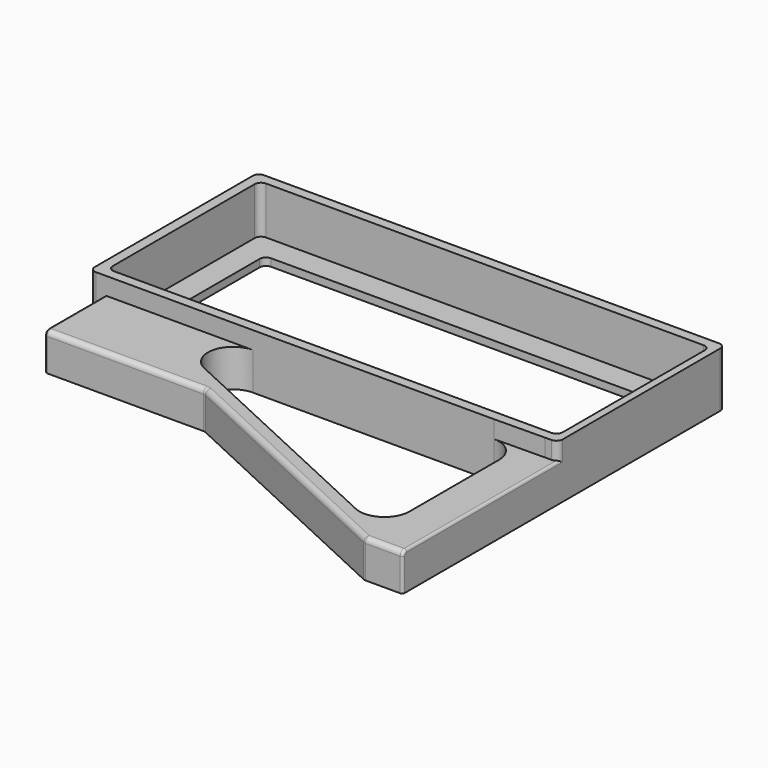
from build123d import *

# Parameters (mm, degrees)
F1_DEPTH     = 22
F2_DEPTH     = 3
F3_DEPTH     = 15
F0_W         = 15
F0_H         = 30
F4_DEPTH     = 15
F5_R         = 2
F6_T1_DEPTH  = 111.1292207426
F6_T3_DEPTH  = 68.4264144678
F6_T5_DEPTH  = 14.1054111362
F6_T10_DEPTH = 2
F6_T14_ANGLE = 24.9330990778
F7_R         = 1
F8_R         = 1
F9_DEPTH     = 5


# Not quite as in the source:
# - a fillet or chamfer that OpenCascade refuses, or shapes differently, is made with other operations: its cross-section is extruded or revolved along the edge and cut away or added
# - a feature names something its author has since deleted; it is built from what else it names


with BuildPart() as f1:
    # F0 (on Top) → F1 (new body)
    with BuildSketch(Plane.XY):
        with BuildLine():
            ThreePointArc((93, 77.5), (92.267766953, 79.267766953), (90.5, 80))
            Line((90.5, 80), (36.5, 80))
            Line((36.5, 80), (24.5, 80))
            Line((24.5, 80), (19, 80))
            Line((19, 80), (-7, 80))
            Line((-7, 80), (-12.5, 80))
            Line((-12.5, 80), (-24.5, 80))
            Line((-24.5, 80), (-74, 80))
            Line((-74, 80), (-91.5, 80))
            ThreePointArc((-91.5, 80), (-93.267766953, 79.267766953), (-94, 77.5))
            Line((-94, 77.5), (-94, 76))
            Line((-94, 76), (-94, 0))
            Line((-94, 0), (-94, -1.5))
            ThreePointArc((-94, -1.5), (-93.267766953, -3.267766953), (-91.5, -4))
            Line((-91.5, -4), (-88, -4))
            Line((-88, -4), (-73, -4))
            Line((-73, -4), (-28.6959191337, -4))
            Line((-28.6959191337, -4), (67.7072161436, -4))
            Line((67.7072161436, -4), (88, -3.7670015892))
            Line((88, -3.7670015892), (90.5, -3.7670015892))
            ThreePointArc((90.5, -3.7670015892), (92.267766953, -3.0347685421), (93, -1.2670015892))
            Line((93, -1.2670015892), (93, 0))
            Line((93, 0), (93, 76))
            Line((93, 76), (93, 77.5))
        make_face()
        with BuildLine():
            ThreePointArc((90, 2.5), (89.267766953, 0.732233047), (87.5, 0))
            Line((87.5, 0), (-87.5, 0))
            ThreePointArc((-87.5, 0), (-89.267766953, 0.732233047), (-90, 2.5))
            Line((-90, 2.5), (-90, 73.5))
            ThreePointArc((-90, 73.5), (-89.267766953, 75.267766953), (-87.5, 76))
            Line((-87.5, 76), (87.5, 76))
            ThreePointArc((87.5, 76), (89.267766953, 75.267766953), (90, 73.5))
            Line((90, 73.5), (90, 2.5))
        make_face(mode=Mode.SUBTRACT)
    extrude(amount=F1_DEPTH)

    # F0 (on Top) → F2 (join)
    with BuildSketch(Plane.XY):
        with BuildLine():
            Line((-87.5, 0), (87.5, 0))
            ThreePointArc((87.5, 0), (89.267766953, 0.732233047), (90, 2.5))
            Line((90, 2.5), (90, 73.5))
            ThreePointArc((90, 73.5), (89.267766953, 75.267766953), (87.5, 76))
            Line((87.5, 76), (-87.5, 76))
            ThreePointArc((-87.5, 76), (-89.267766953, 75.267766953), (-90, 73.5))
            Line((-90, 73.5), (-90, 2.5))
            ThreePointArc((-90, 2.5), (-89.267766953, 0.732233047), (-87.5, 0))
        make_face()
        with BuildLine():
            Line((-77.5, 66), (77.5, 66))
            ThreePointArc((77.5, 66), (79.267766953, 65.267766953), (80, 63.5))
            Line((80, 63.5), (80, 12.5))
            ThreePointArc((80, 12.5), (79.267766953, 10.732233047), (77.5, 10))
            Line((77.5, 10), (-77.5, 10))
            ThreePointArc((-77.5, 10), (-79.267766953, 10.732233047), (-80, 12.5))
            Line((-80, 12.5), (-80, 63.5))
            ThreePointArc((-80, 63.5), (-79.267766953, 65.267766953), (-77.5, 66))
        make_face(mode=Mode.SUBTRACT)
    extrude(amount=F2_DEPTH)

    # F0 (on Top) → F3 (join)
    with BuildSketch(Plane.XY):
        with BuildLine():
            Line((93, -81.2670015892), (93, -1.2670015892))
            ThreePointArc((93, -1.2670015892), (92.267766953, -3.0347685421), (90.5, -3.7670015892))
            Line((90.5, -3.7670015892), (88, -3.7670015892))
            Line((88, -3.7670015892), (67.7072161436, -4))
            ThreePointArc((67.7072161436, -4), (74.7782839555, -6.9289321881), (77.7072161436, -14))
            Line((77.7072161436, -14), (77.7072161436, -58.7379819401))
            ThreePointArc((77.7072161436, -58.7379819401), (73.0879609173, -67.1669549309), (63.4976990076, -67.8088124137))
            Line((63.4976990076, -67.8088124137), (-32.9054362697, -23.0708304737))
            ThreePointArc((-32.9054362697, -23.0708304737), (-38.4608642113, -11.8445771571), (-28.6959191337, -4))
            Line((-28.6959191337, -4), (-73, -4))
            Line((-73, -4), (-73, -34))
            Line((-73, -34), (-24.5735855322, -34))
            ThreePointArc((-24.5735855322, -34), (-24.033911544, -34.0589444934), (-23.5196862036, -34.2329984108))
            Line((-23.5196862036, -34.2329984108), (77.653316815, -81.2670015892))
            Line((77.653316815, -81.2670015892), (93, -81.2670015892))
        make_face()
    extrude(amount=F3_DEPTH)

    # F0 (on Top) → F4 (join)
    with BuildSketch(Plane.XY):
        with Locations((-80.5, -19)):
            Rectangle(F0_W, F0_H)
    extrude(amount=F4_DEPTH)

    # F5
    f5_edges = [f1.edges().sort_by_distance(p)[0] for p in [
        (85.326658, -81.267002, 15),
    ]]
    fillet(f5_edges, radius=F5_R)

    # F6: fillet of radius 2 on 4 edges, made by hand

    # F6_s2 → F6_t1 (cut)
    with BuildSketch(Plane(origin=(-6.2536714965, 2.9072499211, 0), x_dir=(0, 0, 1), z_dir=(0.9068006357, -0.4215597314, 0))):
        with BuildLine():
            ThreePointArc((15, 38.9574573188), (14.4142135624, 40.3716708812), (13, 40.9574573188))
            Line((13, 40.9574573188), (15, 40.9574573188))
            Line((15, 40.9574573188), (15, 38.9574573188))
        make_face()
    extrude(amount=F6_T1_DEPTH, mode=Mode.SUBTRACT)

    # F6_s4 → F6_t3 (cut)
    with BuildSketch(Plane.YZ.offset(-93)):
        with BuildLine():
            ThreePointArc((-32, 15), (-33.4142135624, 14.4142135624), (-34, 13))
            Line((-34, 13), (-34, 15))
            Line((-34, 15), (-32, 15))
        make_face()
    extrude(amount=F6_T3_DEPTH, mode=Mode.SUBTRACT)

    # F6_s6 → F6_t5 (cut)
    with BuildSketch(Plane.XY.offset(-1.1054111362)):
        with BuildLine():
            ThreePointArc((77.2523618067, -81.0806028605), (77.6637420789, -81.2198459945), (78.0954812695, -81.2670015892))
            Line((78.0954812695, -81.2670015892), (77.653316815, -81.2670015892))
            Line((77.653316815, -81.2670015892), (77.2523618067, -81.0806028605))
        make_face()
    extrude(amount=F6_T5_DEPTH, mode=Mode.SUBTRACT)


with BuildPart() as f6_tool8:
    # F6_s9 → F6_t10 (new body)
    with BuildSketch(Plane.XY.offset(13)):
        Polygon((78.0954812695, -79.2670015892), (78.0954812695, -81.2670015892), (77.653316815, -81.2670015892), (77.2523618067, -81.0806028605), align=None)
    extrude(amount=F6_T10_DEPTH)

    # F6_s11 → F6_t12 (revolve, cut)
    with BuildSketch(Plane(origin=(78.0954812695, -79.2670015892, 13), x_dir=(0.2158695953, 0.9764222027, 0), z_dir=(0.9764222027, -0.2158695953, 0))):
        with BuildLine():
            ThreePointArc((0, -2), (2, 0), (0, 2))
            Line((0, 2), (0, -2))
        make_face()
    revolve(axis=Axis((78.0954812695, -79.2670015892, 13), (0, 0, 1)), mode=Mode.SUBTRACT)


with BuildPart() as f1_1:
    add(f1.part)

    # F6_t7: cut F6_tool8
    add(f6_tool8.part, mode=Mode.SUBTRACT)

    # F6_s13 → F6_t14 (revolve, cut)
    with BuildSketch(Plane.YZ.offset(-24.5735855322)):
        with BuildLine():
            ThreePointArc((-32, 15), (-33.4142135624, 14.4142135624), (-34, 13))
            Line((-34, 13), (-34, 15))
            Line((-34, 15), (-32, 15))
        make_face()
    revolve(axis=Axis((-24.5735855322, -36.5, 15), (0, 0, -1)), revolution_arc=F6_T14_ANGLE, mode=Mode.SUBTRACT)

    # F7
    f7_edges = [f1_1.edges().sort_by_distance(p)[0] for p in [
        (93, -81.267002, 6.5),
    ]]
    fillet(f7_edges, radius=F7_R)

    # F8
    f8_edges = [f1_1.edges().sort_by_distance(p)[0] for p in [
        (-88, -34, 6.5),
        (-88, -18, 15),
        (-88, -33.414214, 14.414214),
    ]]
    fillet(f8_edges, radius=F8_R)

    # F0 (on Top) → F9 (join)
    with BuildSketch(Plane.XY):
        with BuildLine():
            Line((-24.5, 80), (-12.5, 80))
            Line((-12.5, 80), (-12.5, 89.5))
            ThreePointArc((-12.5, 89.5), (-13.232233047, 91.267766953), (-15, 92))
            Line((-15, 92), (-22, 92))
            ThreePointArc((-22, 92), (-23.767766953, 91.267766953), (-24.5, 89.5))
            Line((-24.5, 89.5), (-24.5, 80))
        make_face()
        with BuildLine():
            Line((-7, 80), (19, 80))
            Line((19, 80), (19, 89.5))
            ThreePointArc((19, 89.5), (18.267766953, 91.267766953), (16.5, 92))
            Line((16.5, 92), (-4.5, 92))
            ThreePointArc((-4.5, 92), (-6.267766953, 91.267766953), (-7, 89.5))
            Line((-7, 89.5), (-7, 80))
        make_face()
        with BuildLine():
            Line((24.5, 80), (36.5, 80))
            Line((36.5, 80), (36.5, 89.5))
            ThreePointArc((36.5, 89.5), (35.767766953, 91.267766953), (34, 92))
            Line((34, 92), (27, 92))
            ThreePointArc((27, 92), (25.232233047, 91.267766953), (24.5, 89.5))
            Line((24.5, 89.5), (24.5, 80))
        make_face()
    extrude(amount=F9_DEPTH)


solid = f1_1.part
